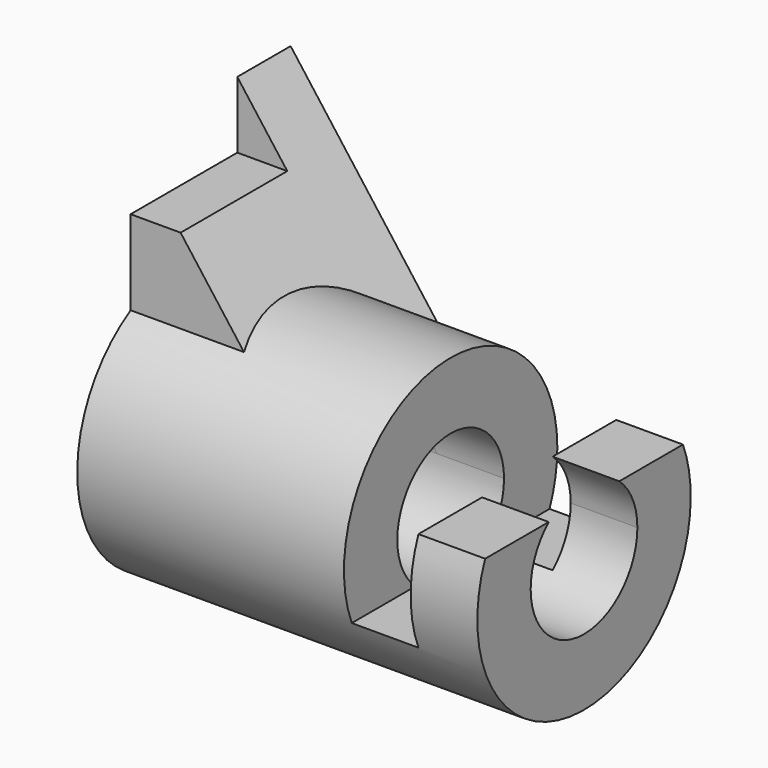
from build123d import *
from build123d import SkipClean  # not in build123d's __all__

# Parameters (mm, degrees)
F1_DEPTH  = 38.1
F4_DEPTH  = 38.1
F2_R      = 25.4
F2_R_2    = 12.7
F5_DEPTH  = 76.2
F6_W      = 23.5464301965
F6_H      = 15.875
F7_DEPTH  = 25.4
F9_DEPTH  = 19.05
F11_R     = 12.7
F12_DEPTH = 76.201


# Not quite as in the source:
# - a feature of the source that left no trace in its solid (it failed there, or was rolled back) is left out


with BuildPart() as f1:
    # F0 (on Right) → F1 (new body)
    with BuildSketch(Plane.YZ):
        Polygon((-12.7, 0), (0, 0), (25.4, 0), (25.4, 50.8), (12.7, 50.8), (12.7, 38.1), (0, 38.1), (-12.7, 38.1), align=None)
    extrude(amount=F1_DEPTH)

    # F3 (on face) → F4 (cut)
    with BuildSketch(Plane(origin=(0, 25.4, 0), x_dir=(-1, 0, 0), z_dir=(0, 1, 0))):
        Polygon((-38.1, 50.8), (-38.1, 0), (0, 50.8), align=None)
    extrude(amount=-F4_DEPTH, mode=Mode.SUBTRACT)

    # F2 (on Right) → F5 (join)
    with BuildSketch(Plane.YZ):
        Circle(F2_R)
        Circle(F2_R_2, mode=Mode.SUBTRACT)
    extrude(amount=F5_DEPTH)

    # F6 (on face) → F7 (cut)
    with BuildSketch(Plane.YZ.offset(76.2)):
        with Locations((11.7732150983, 17.4625)):
            Rectangle(F6_W, F6_H)
        with Locations((-11.7732150983, 17.4625)):
            Rectangle(F6_W, F6_H)
    extrude(amount=-F7_DEPTH, mode=Mode.SUBTRACT)

    # F8 (on face) → F9 (cut)
    with BuildSketch(Plane.XY.offset(9.525)):
        Polygon((63.5, -27.7675297111), (63.5, 8.4002604126), (63.5, 27.7675297111), (50.8, 27.7675297111), (50.8, -27.7675297111), align=None)
    extrude(amount=-F9_DEPTH, mode=Mode.SUBTRACT)

    # F11 (on face) → F12 (cut, through all)
    with BuildSketch(Plane(origin=(0, 0, 0), x_dir=(0, -1, 0), z_dir=(-1, 0, 0))):
        Circle(F11_R)
    with SkipClean():  # cleaning this boolean's faces spoils the solid; the shape is the same uncleaned
        extrude(amount=-F12_DEPTH, mode=Mode.SUBTRACT)


solid = f1.part
